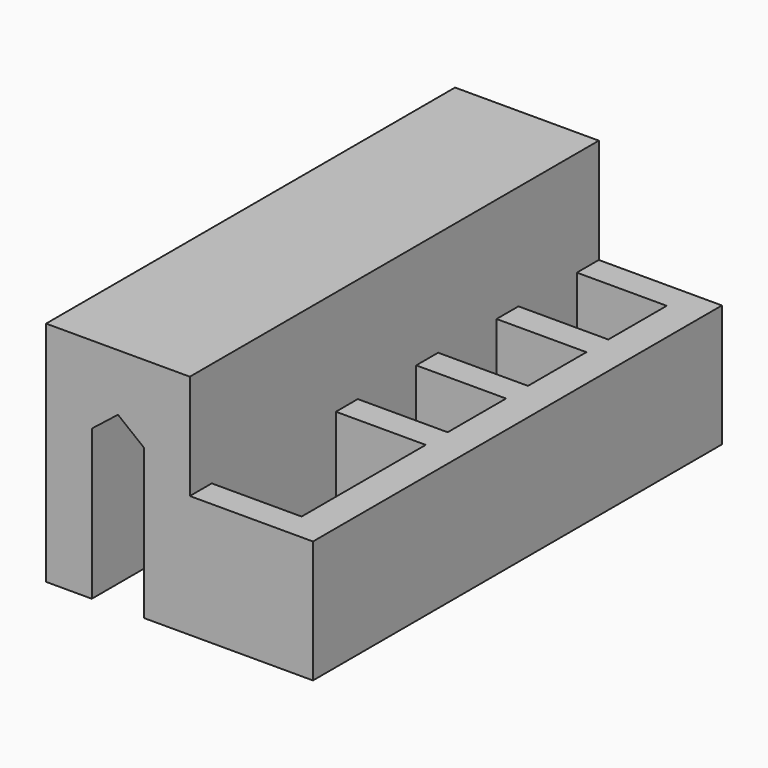
from build123d import *

# Parameters (mm, degrees)
F0_W     = 0.026536879
F0_H     = 8.3333357554
F0_W_2   = 14.573463121
F1_DEPTH = 142.24
F2_W     = 27.8897660319
F2_H     = 8.4373559803
F3_DEPTH = 2.54
F4_W     = 25
F4_H     = 7.62
F5_DEPTH = 25.4


with BuildPart() as f1:
    # F0 (on Front) → F1 (new body)
    with BuildSketch(Plane.XZ):
        Polygon((-54.4296333165, 41.6801715141), (-54.4296333165, 16.0493828058), (-67.1296333165, 16.0493828058), (-67.1296333165, 0), (-54.4030964375, 0), (-54.4030964375, 41.7011594015), align=None)
        Polygon((-67.1296333165, 16.0493828058), (-54.4296333165, 16.0493828058), (-54.4296333165, 41.6801715141), (-67.1296333165, 31.6358038057), align=None)
        Polygon((-67.1296333165, 31.6358038057), (-54.4296333165, 41.6801715141), (-54.4296333165, 53.2272399031), (-56.5930453334, 54.9382718561), (-67.1296333165, 54.9382718561), align=None)
        Polygon((-54.4296333165, 53.2272399031), (-54.4296333165, 41.6801715141), (-54.4030964375, 41.7011594015), (-54.4030964375, 53.2062520157), align=None)
        Polygon((-56.5930453334, 54.9382718561), (-54.4296333165, 53.2272399031), (-54.4296333165, 54.9382718561), align=None)
        Polygon((-54.4296333165, 54.9382718561), (-54.4296333165, 53.2272399031), (-54.4030964375, 53.2062520157), (-54.4030964375, 54.9382718561), align=None)
        Polygon((-54.4030964375, 53.2062520157), (-54.4030964375, 41.7011594015), (-47.1296333165, 47.4537057086), align=None)
        Polygon((-67.1296333165, 63.2716076115), (-67.1296333165, 54.9382718561), (-56.5930453334, 54.9382718561), align=None)
        Polygon((-56.5930453334, 54.9382718561), (-54.4296333165, 54.9382718561), (-54.4296333165, 63.2716076115), (-67.1296333165, 63.2716076115), align=None)
        with Locations((-54.416364877, 59.1049397338)):
            Rectangle(F0_W, F0_H)
        Polygon((-54.4030964375, 54.9382718561), (-54.4030964375, 53.2062520157), (-47.1296333165, 47.4537057086), (-39.8296333165, 53.2272399031), (-39.8296333165, 54.9382718561), align=None)
        Polygon((-39.8296333165, 53.2272399031), (-47.1296333165, 47.4537057086), (-39.8296333165, 41.6801715141), align=None)
        with Locations((-47.116364877, 59.1049397338)):
            Rectangle(F0_W_2, F0_H)
        Polygon((-37.6662212996, 54.9382718561), (-39.8296333165, 53.2272399031), (-39.8296333165, 41.6801715141), (-27.1296333165, 31.6358038057), (-27.1296333165, 54.9382718561), align=None)
        Polygon((-39.8296333165, 54.9382718561), (-39.8296333165, 53.2272399031), (-37.6662212996, 54.9382718561), align=None)
        Polygon((-27.1296333165, 31.6358038057), (-39.8296333165, 41.6801715141), (-39.8296333165, 8.6419750216), (-39.8296333165, 0), (-27.1296333165, 0), (-27.1296333165, 8.6419750216), align=None)
        Polygon((-39.8296333165, 63.2716076115), (-39.8296333165, 54.9382718561), (-37.6662212996, 54.9382718561), (-27.1296333165, 63.2716076115), align=None)
        Polygon((-27.1296333165, 63.2716076115), (-37.6662212996, 54.9382718561), (-27.1296333165, 54.9382718561), align=None)
        Polygon((-2.1296333165, 8.6419750216), (-27.1296333165, 8.6419750216), (-27.1296333165, 0), (-2.1296333165, 0), (-2.1296333165, 1.0219750216), align=None)
        Polygon((-2.1296333165, 34.0419750216), (-2.1296333165, 8.6419750216), (-2.1296333165, 1.0219750216), (-2.1296333165, 0), (7.1296278669, 0), (7.1296278669, 1.0219750216), (7.1296278669, 34.0419750216), align=None)
    extrude(amount=F1_DEPTH)

    # F2 (on face) → F3 (join)
    with BuildSketch(Plane.XZ.offset(142.24)):
        with Locations((-25.8847503005, 4.2186779901)):
            Rectangle(F2_W, F2_H)
    extrude(amount=-F3_DEPTH)

    # F4 (on face) → F5 (join)
    with BuildSketch(Plane.XY.offset(8.6419750216)):
        with Locations((-14.6296333165, -87.63)):
            Rectangle(F4_W, F4_H)
        with Locations((-14.6296333165, -59.69)):
            Rectangle(F4_W, F4_H)
        with Locations((-14.6296333165, -31.75)):
            Rectangle(F4_W, F4_H)
        with Locations((-14.6296333165, -3.81)):
            Rectangle(F4_W, F4_H)
        Polygon((-2.1296333165, -139.7), (-2.1296333165, -134.62), (-27.1296333165, -134.62), (-27.1296333165, -142.24), (-2.1296333165, -142.24), align=None)
    extrude(amount=F5_DEPTH)


solid = f1.part
